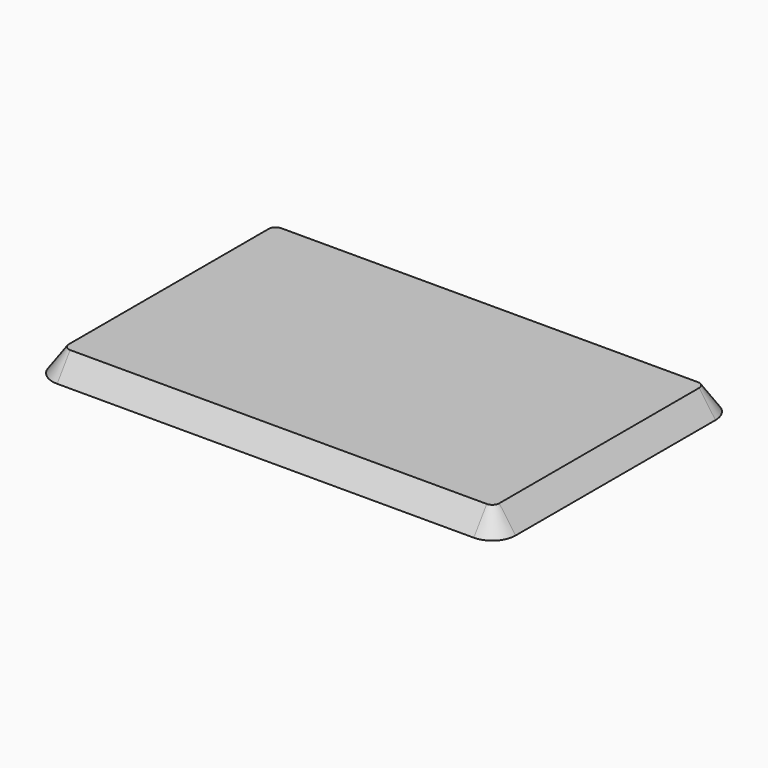
from build123d import *

# Parameters (mm, degrees)
F0_W     = 50
F0_H     = 32
F1_DEPTH = 2.5
F2_R     = 2.5
F3_SIZE2 = 2.49999
F3_SIZE  = 1.750509


# Not quite as in the source:
# - a fillet or chamfer is up to 0.001 mm smaller than in the source, because OpenCascade refuses the exact size


with BuildPart() as f1:
    # F0 (on Top) → F1 (new body)
    with BuildSketch(Plane.XY):
        Rectangle(F0_W, F0_H)
    extrude(amount=F1_DEPTH)

    # F2
    f2_edges = [f1.edges().sort_by_distance(p)[0] for p in [
        (-25, -16, 1.25),
        (25, -16, 1.25),
        (25, 16, 1.25),
        (-25, 16, 1.25),
    ]]
    fillet(f2_edges, radius=F2_R)

    # F3 (size 1.7505188455 and 2.5 in the source; OpenCascade refuses exactly that, so slightly less here)
    f3_edges = [f1.edges().sort_by_distance(p)[0] for p in [
        (0, -16, 2.5),
        (-24.267767, -15.267767, 2.5),
        (-25, 0, 2.5),
        (-24.267767, 15.267767, 2.5),
        (0, 16, 2.5),
        (24.267767, 15.267767, 2.5),
        (25, 0, 2.5),
        (24.267767, -15.267767, 2.5),
    ]]
    f3_side = f1.faces().sort_by_distance((0, 0, 2.5))[0]
    chamfer(f3_edges, length=F3_SIZE, length2=F3_SIZE2, reference=f3_side)


solid = f1.part
